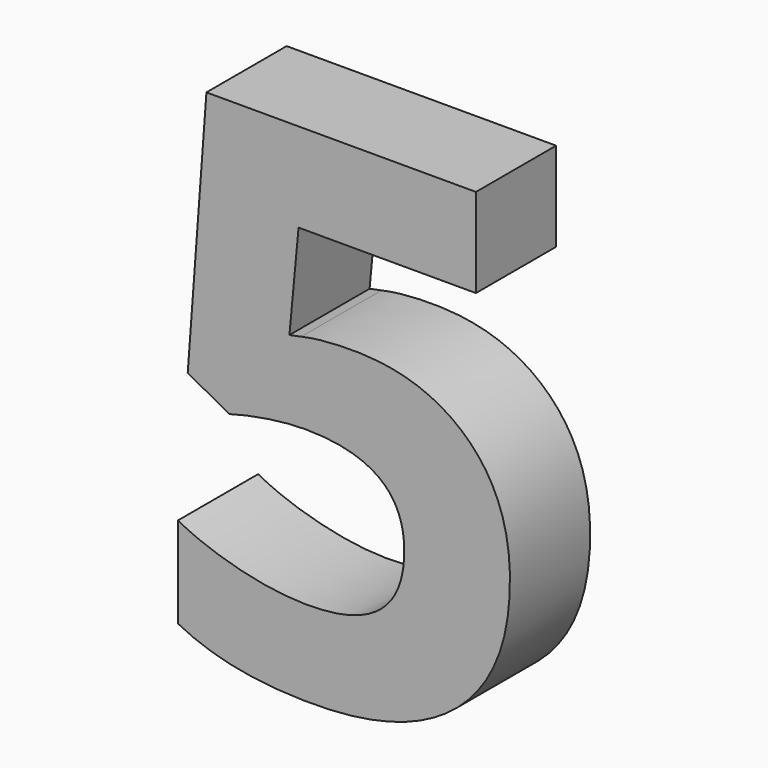
from build123d import *

# Parameters (mm, degrees)
F0_TEXT_SIZE = 35.2777777778
F1_DEPTH     = 5.08


# Not quite as in the source:
# - Text() gives the source's letters only with a copy of the font that has no kerning and outlines rounded to 1/6400 em; it was checked with that copy


with BuildPart() as f1:
    # F0 (on Front) → F1 (new body)
    with BuildSketch(Plane.XZ):
        with Locations((-91.5053262118, -14.3813476095)):
            Text('5', F0_TEXT_SIZE, font='Open Sans', font_style=FontStyle.BOLD, text_align=(TextAlign.LEFT, TextAlign.BOTTOM))
    extrude(amount=F1_DEPTH)


solid = f1.part
